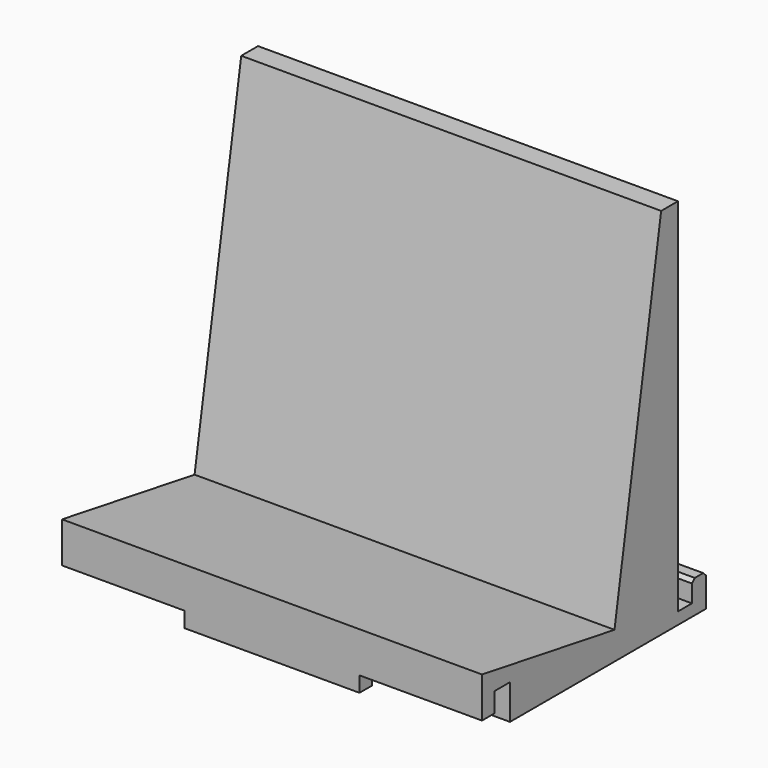
from build123d import *

# Parameters (mm, degrees)
F0_W      = 60
F0_H      = 40
F1_DEPTH  = 4
F3_DEPTH  = 60
F4_W      = 2.2
F4_H      = 2.2
F4_W_2    = 2.5
F4_H_2    = 2.3
F5_DEPTH  = 60
F4_H_3    = 0.7
F6_DEPTH  = 60
F7_W      = 25
F7_H      = 2.2
F8_DEPTH  = 2.2
F9_W      = 26
F9_H      = 2.5
F10_DEPTH = 1.7
F11_SIZE  = 0.5


with BuildPart() as f1:
    # F0 (on Top) → F1 (new body)
    with BuildSketch(Plane.XY):
        Rectangle(F0_W, F0_H)
    extrude(amount=F1_DEPTH)

    # F2 (on face) → F3 (join, through all)
    with BuildSketch(Plane.YZ.offset(30)):
        Polygon((12, 53.300871376), (3.6678885292, 4), (15, 4), (15, 53.300871376), align=None)
        Polygon((-20, 8), (-20, 4), (3.6678885292, 4), align=None)
    extrude(amount=-F3_DEPTH)

    # F4 (on face) → F5 (cut, through all)
    with BuildSketch(Plane.YZ.offset(30)):
        with Locations((-18.9, 1.1)):
            Rectangle(F4_W, F4_H)
        Polygon((-17.8, 2.2), (-17.8, 0), (-15, 0), (-15, 5), (-17.8, 5), align=None)
        with Locations((16.25, 2.85)):
            Rectangle(F4_W_2, F4_H_2)
    extrude(amount=-F5_DEPTH, mode=Mode.SUBTRACT)

    # F4 (on face) → F6 (join, through all)
    with BuildSketch(Plane.YZ.offset(30)):
        with Locations((18.75, 4.35)):
            Rectangle(F4_W_2, F4_H_3)
    extrude(amount=-F6_DEPTH)

    # F7 (on face) → F8 (join, through all)
    with BuildSketch(Plane(origin=(0, 0, 2.2), x_dir=(1, 0, 0), z_dir=(0, 0, -1))):
        with Locations((0, 18.9)):
            Rectangle(F7_W, F7_H)
    extrude(amount=F8_DEPTH)

    # F9 (on face) → F10 (cut, through all)
    with BuildSketch(Plane.XY.offset(1.7)):
        with Locations((0, 16.25)):
            Rectangle(F9_W, F9_H)
    extrude(amount=-F10_DEPTH, mode=Mode.SUBTRACT)

    # F11
    f11_edges = [f1.edges().sort_by_distance(p)[0] for p in [
        (0, 20, 4.7),
        (0, 17.5, 4.7),
        (-13, 16.25, 1.7),
        (13, 16.25, 1.7),
    ]]
    chamfer(f11_edges, length=F11_SIZE)


solid = f1.part
